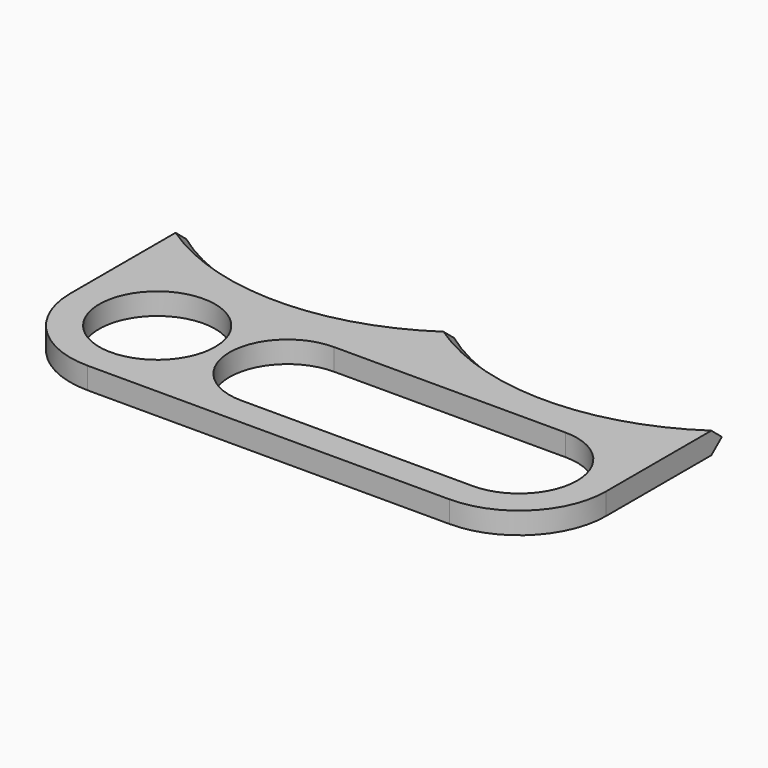
from build123d import *

# Parameters (mm, degrees)
F0_R     = 12.7
F1_DEPTH = 4.7625
F2_SIZE  = 2.38124


# Not quite as in the source:
# - a fillet or chamfer is up to 0.001 mm smaller than in the source, because OpenCascade refuses the exact size


with BuildPart() as f1:
    # F0 (on Top) → F1 (new body)
    with BuildSketch(Plane.XY):
        with BuildLine():
            Line((-19.05, 31.75), (-19.05, 0))
            ThreePointArc((-19.05, 0), (-13.4703841816, -13.4703841816), (0, -19.05))
            Line((0, -19.05), (79.375, -19.05))
            ThreePointArc((79.375, -19.05), (92.8453841816, -13.4703841816), (98.425, 0))
            Line((98.425, 0), (98.425, 31.75))
            ThreePointArc((98.425, 31.75), (69.05625, 22.225), (39.6875, 31.75))
            ThreePointArc((39.6875, 31.75), (10.31875, 22.225), (-19.05, 31.75))
        make_face()
        Circle(F0_R, mode=Mode.SUBTRACT)
        with BuildLine():
            Line((79.375, -12.7), (28.575, -12.7))
            ThreePointArc((28.575, -12.7), (15.875, 0), (28.575, 12.7))
            Line((28.575, 12.7), (79.375, 12.7))
            ThreePointArc((79.375, 12.7), (92.075, 0), (79.375, -12.7))
        make_face(mode=Mode.SUBTRACT)
    extrude(amount=F1_DEPTH)

    # F2 (size 2.38125 in the source; OpenCascade refuses exactly that, so slightly less here)
    f2_edges = [f1.edges().sort_by_distance(p)[0] for p in [
        (10.31875, 22.225, 4.7625),
        (69.05625, 22.225, 4.7625),
        (69.05625, 22.225, 0),
        (10.31875, 22.225, 0),
    ]]
    chamfer(f2_edges, length=F2_SIZE)


solid = f1.part
